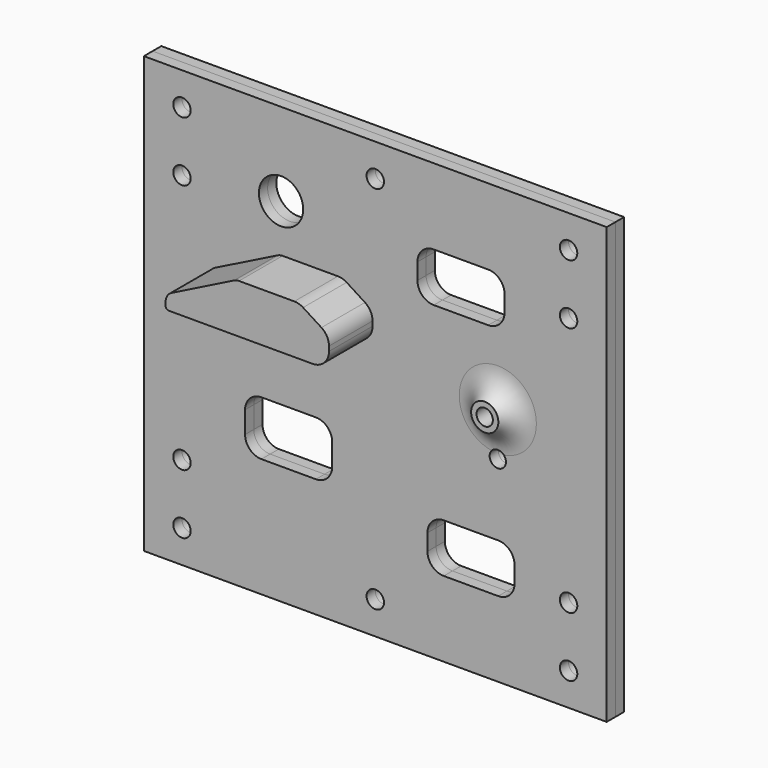
from build123d import *

# Parameters (mm, degrees)
F0_R          = 2.5
F0_R_2        = 1.6
F0_R_3        = 1.5
F1_DEPTH      = 2
F3_DEPTH      = 10
F4_DEPTH      = 3
F4_DEPTH_BACK = 2
F5_S5_R       = 1.5
F5_T6_DEPTH   = 13
F6_R          = 4.0661391715
F7_DEPTH      = 25


# Not quite as in the source:
# - a fillet or chamfer that OpenCascade refuses, or shapes differently, is made with other operations: its cross-section is extruded or revolved along the edge and cut away or added


with BuildPart() as f1:
    # F0 (on Front) → F1 (new body)
    with BuildSketch(Plane.XZ):
        Polygon((42.5, -4), (42.5, 4), (42.5, 6), (-42.5, 6), (-42.5, 4), (-42.5, -4), (-42.5, -34), (42.5, -34), align=None)
        with BuildLine():
            Line((-3.5, -27), (-29.945935972, -27))
            ThreePointArc((-29.945935972, -27), (-30.3377184034, -26.8377184034), (-30.5, -26.445935972))
            Line((-30.5, -26.445935972), (-30.5, -25.7360679775))
            ThreePointArc((-30.5, -25.7360679775), (-30.2013016167, -24.6846057533), (-29.394427191, -23.9472135955))
            Line((-29.394427191, -23.9472135955), (-17.922291236, -18.211145618))
            ThreePointArc((-17.922291236, -18.211145618), (-17.4873698861, -18.0535020211), (-17.027864045, -18))
            Line((-17.027864045, -18), (-6.8736020616, -18))
            ThreePointArc((-6.8736020616, -18), (-6.0348391003, -18.1196394853), (-5.262975585, -18.4690155368))
            Line((-5.262975585, -18.4690155368), (-1.8893735234, -20.6158532124))
            ThreePointArc((-1.8893735234, -20.6158532124), (-0.87018257, -21.7032102011), (-0.5, -23.1468376756))
            Line((-0.5, -23.1468376756), (-0.5, -24))
            ThreePointArc((-0.5, -24), (-1.3786796564, -26.1213203436), (-3.5, -27))
        make_face(mode=Mode.SUBTRACT)
        with Locations((22.5, -30)):
            Circle(F0_R, mode=Mode.SUBTRACT)
        with Locations((-35.5, -11)):
            Circle(F0_R_2, mode=Mode.SUBTRACT)
        with Locations((-35.5, 0)):
            Circle(F0_R_2, mode=Mode.SUBTRACT)
        with Locations((35.5, -11)):
            Circle(F0_R_2, mode=Mode.SUBTRACT)
        Circle(F0_R_2, mode=Mode.SUBTRACT)
        with Locations((35.5, 0)):
            Circle(F0_R_2, mode=Mode.SUBTRACT)
        with BuildLine():
            ThreePointArc((-30.5, -26.445935972), (-30.3377184034, -26.8377184034), (-29.945935972, -27))
            Line((-29.945935972, -27), (-3.5, -27))
            ThreePointArc((-3.5, -27), (-1.3786796564, -26.1213203436), (-0.5, -24))
            Line((-0.5, -24), (-0.5, -23.1468376756))
            ThreePointArc((-0.5, -23.1468376756), (-0.87018257, -21.7032102011), (-1.8893735234, -20.6158532124))
            Line((-1.8893735234, -20.6158532124), (-5.262975585, -18.4690155368))
            ThreePointArc((-5.262975585, -18.4690155368), (-6.0348391003, -18.1196394853), (-6.8736020616, -18))
            Line((-6.8736020616, -18), (-17.027864045, -18))
            ThreePointArc((-17.027864045, -18), (-17.4873698861, -18.0535020211), (-17.922291236, -18.211145618))
            Line((-17.922291236, -18.211145618), (-29.394427191, -23.9472135955))
            ThreePointArc((-29.394427191, -23.9472135955), (-30.2013016167, -24.6846057533), (-30.5, -25.7360679775))
            Line((-30.5, -25.7360679775), (-30.5, -26.445935972))
        make_face()
        with Locations((22.5, -30)):
            Circle(F0_R)
        with Locations((22.5, -30)):
            Circle(F0_R_3, mode=Mode.SUBTRACT)
    extrude(amount=-F1_DEPTH)

    # F2: F1 across face


with BuildPart() as f1_1:
    add(f1.part)
    add(f1.part.mirror(Plane(origin=(0, 1, -34), x_dir=(1, 0, 0), z_dir=(0, 0, -1))))

    # F0 (on Front) → F3 (join)
    with BuildSketch(Plane.XZ):
        with BuildLine():
            ThreePointArc((-30.5, -26.445935972), (-30.3377184034, -26.8377184034), (-29.945935972, -27))
            Line((-29.945935972, -27), (-3.5, -27))
            ThreePointArc((-3.5, -27), (-1.3786796564, -26.1213203436), (-0.5, -24))
            Line((-0.5, -24), (-0.5, -23.1468376756))
            ThreePointArc((-0.5, -23.1468376756), (-0.87018257, -21.7032102011), (-1.8893735234, -20.6158532124))
            Line((-1.8893735234, -20.6158532124), (-5.262975585, -18.4690155368))
            ThreePointArc((-5.262975585, -18.4690155368), (-6.0348391003, -18.1196394853), (-6.8736020616, -18))
            Line((-6.8736020616, -18), (-17.027864045, -18))
            ThreePointArc((-17.027864045, -18), (-17.4873698861, -18.0535020211), (-17.922291236, -18.211145618))
            Line((-17.922291236, -18.211145618), (-29.394427191, -23.9472135955))
            ThreePointArc((-29.394427191, -23.9472135955), (-30.2013016167, -24.6846057533), (-30.5, -25.7360679775))
            Line((-30.5, -25.7360679775), (-30.5, -26.445935972))
        make_face()
    extrude(amount=F3_DEPTH)

    # F0 (on Front) → F4 (join, two sides)
    with BuildSketch(Plane.XZ) as f4_sk:
        with Locations((22.5, -30)):
            Circle(F0_R)
        with Locations((22.5, -30)):
            Circle(F0_R_3, mode=Mode.SUBTRACT)
    extrude(amount=F4_DEPTH)
    extrude(f4_sk.sketch, amount=-F4_DEPTH_BACK)

    # F5: fillet of radius 5 on 1 edges, made by hand


with BuildPart() as f5_tool2:
    # F5_s3 → F5_t4 (revolve)
    with BuildSketch(Plane.XY.offset(-30)):
        with BuildLine():
            ThreePointArc((29.582575695, 0), (26.8439629074, -0.8166998673), (25, -3))
            Line((25, -3), (25, 0))
            Line((25, 0), (29.582575695, 0))
        make_face()
    revolve(axis=Axis((22.5, 0, -30), (0, -1, 0)))

    # F5_s5 → F5_t6 (cut, symmetric)
    with BuildSketch(Plane.XZ.offset(2.5)):
        with Locations((22.5, -38)):
            Circle(F5_S5_R)
    extrude(amount=F5_T6_DEPTH, both=True, mode=Mode.SUBTRACT)


with BuildPart() as f1_2:
    add(f1_1.part)

    # F5_t1: union F5_tool2
    add(f5_tool2.part)

    # F6 (on face) → F7 (cut)
    with BuildSketch(Plane.XZ):
        with BuildLine():
            Line((22.5772393979, -51.1348243654), (12.5772393979, -51.1348243654))
            ThreePointArc((12.5772393979, -51.1348243654), (10.4559190544, -52.0135040218), (9.5772393979, -54.1348243654))
            Line((9.5772393979, -54.1348243654), (9.5772393979, -57.1348243654))
            ThreePointArc((9.5772393979, -57.1348243654), (10.4559190544, -59.2561447089), (12.5772393979, -60.1348243654))
            Line((12.5772393979, -60.1348243654), (22.5772393979, -60.1348243654))
            ThreePointArc((22.5772393979, -60.1348243654), (24.6985597415, -59.2561447089), (25.5772393979, -57.1348243654))
            Line((25.5772393979, -57.1348243654), (25.5772393979, -54.1348243654))
            ThreePointArc((25.5772393979, -54.1348243654), (24.6985597415, -52.0135040218), (22.5772393979, -51.1348243654))
        make_face()
        with BuildLine():
            Line((-10.9149579704, -42.1334951818), (-20.9149579704, -42.1334951818))
            ThreePointArc((-20.9149579704, -42.1334951818), (-23.0362783139, -43.0121748382), (-23.9149579704, -45.1334951818))
            Line((-23.9149579704, -45.1334951818), (-23.9149579704, -49.1334951818))
            ThreePointArc((-23.9149579704, -49.1334951818), (-23.0362783139, -51.2548155254), (-20.9149579704, -52.1334951818))
            Line((-20.9149579704, -52.1334951818), (-10.9149579704, -52.1334951818))
            ThreePointArc((-10.9149579704, -52.1334951818), (-8.7936376268, -51.2548155254), (-7.9149579704, -49.1334951818))
            Line((-7.9149579704, -49.1334951818), (-7.9149579704, -45.1334951818))
            ThreePointArc((-7.9149579704, -45.1334951818), (-8.7936376268, -43.0121748382), (-10.9149579704, -42.1334951818))
        make_face()
        with BuildLine():
            Line((20.7370246872, -7.9352889061), (10.7370246872, -7.9352889061))
            ThreePointArc((10.7370246872, -7.9352889061), (8.6157043437, -8.8139685625), (7.7370246872, -10.9352889061))
            Line((7.7370246872, -10.9352889061), (7.7370246872, -13.9352889061))
            ThreePointArc((7.7370246872, -13.9352889061), (8.6157043437, -16.0566092497), (10.7370246872, -16.9352889061))
            Line((10.7370246872, -16.9352889061), (20.7370246872, -16.9352889061))
            ThreePointArc((20.7370246872, -16.9352889061), (22.8583450308, -16.0566092497), (23.7370246872, -13.9352889061))
            Line((23.7370246872, -13.9352889061), (23.7370246872, -10.9352889061))
            ThreePointArc((23.7370246872, -10.9352889061), (22.8583450308, -8.8139685625), (20.7370246872, -7.9352889061))
        make_face()
        with Locations((-17.3052940518, -9.25668329)):
            Circle(F6_R)
    extrude(amount=-F7_DEPTH, mode=Mode.SUBTRACT)


with BuildPart() as f8_1:
    # F8: instance of F1
    add(f1_2.part.mirror(Plane(origin=(-0.2465473767, 2, -33.8837241542), x_dir=(-1, 0, 0), z_dir=(0, 1, 0))))


solid = Compound([f1_2.part, f8_1.part])
